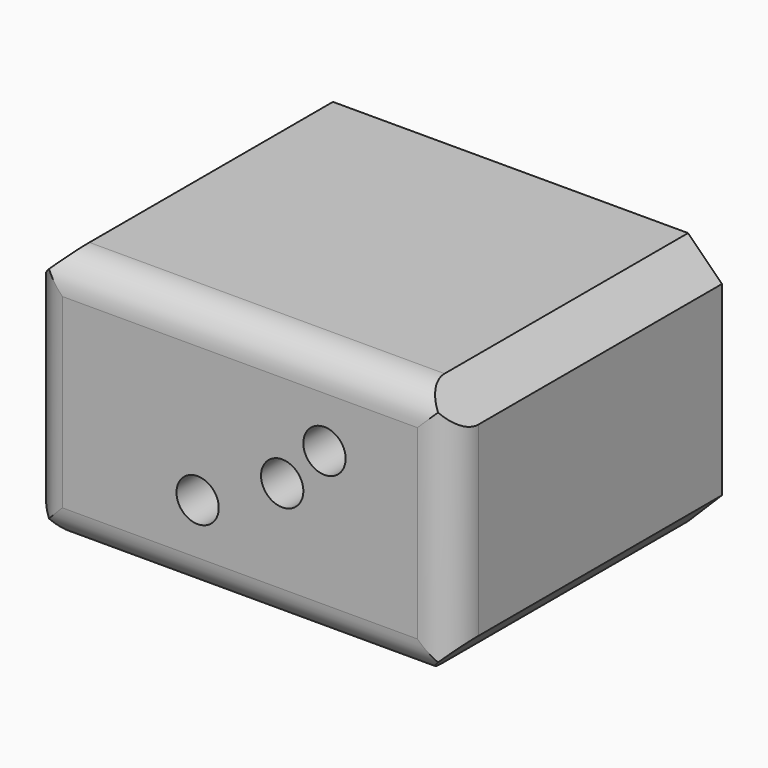
from build123d import *

# Parameters (mm, degrees)
F0_W     = 63.5
F0_H     = 38.1
F1_DEPTH = 50.8
F2_SIZE  = 5.08
F3_R     = 5.08
F3_R_2   = 5.07999
F5_D     = 6.35


# Not quite as in the source:
# - a fillet or chamfer is up to 0.001 mm smaller than in the source, because OpenCascade refuses the exact size


with BuildPart() as f1:
    # F0 (on Front) → F1 (new body)
    with BuildSketch(Plane.XZ):
        with Locations((31.75, 19.05)):
            Rectangle(F0_W, F0_H)
    extrude(amount=-F1_DEPTH)

    # F2
    f2_edges = [f1.edges().sort_by_distance(p)[0] for p in [
        (63.5, 25.4, 38.1),
        (0, 25.4, 38.1),
        (63.5, 25.4, 0),
        (0, 25.4, 0),
    ]]
    chamfer(f2_edges, length=F2_SIZE)

    # F3 (call 1 of 4: OpenCascade refuses the feature's edges together)
    f3_edges = [f1.edges().sort_by_distance(p)[0] for p in [
        (63.5, 0, 19.05),
    ]]
    fillet(f3_edges, radius=F3_R)

    # F3#2 (call 2 of 4)
    f3_2_edges = [f1.edges().sort_by_distance(p)[0] for p in [
        (0, 0, 19.05),
    ]]
    fillet(f3_2_edges, radius=F3_R)

    # F3#3 (call 3 of 4) (radius 5.08 in the source; OpenCascade refuses exactly that, so slightly less here)
    f3_3_edges = [f1.edges().sort_by_distance(p)[0] for p in [
        (31.75, 0, 0),
    ]]
    fillet(f3_3_edges, radius=F3_R_2)

    # F3#4 (call 4 of 4) (radius 5.08 in the source; OpenCascade refuses exactly that, so slightly less here)
    f3_4_edges = [f1.edges().sort_by_distance(p)[0] for p in [
        (31.75, 0, 38.1),
    ]]
    fillet(f3_4_edges, radius=F3_R_2)

    # F5 (through all)
    with Locations(Plane.XZ):
        with Locations((25.4, 12.7), (44.45, 25.4), (38.1, 19.05)):
            Hole(F5_D / 2)


solid = f1.part
